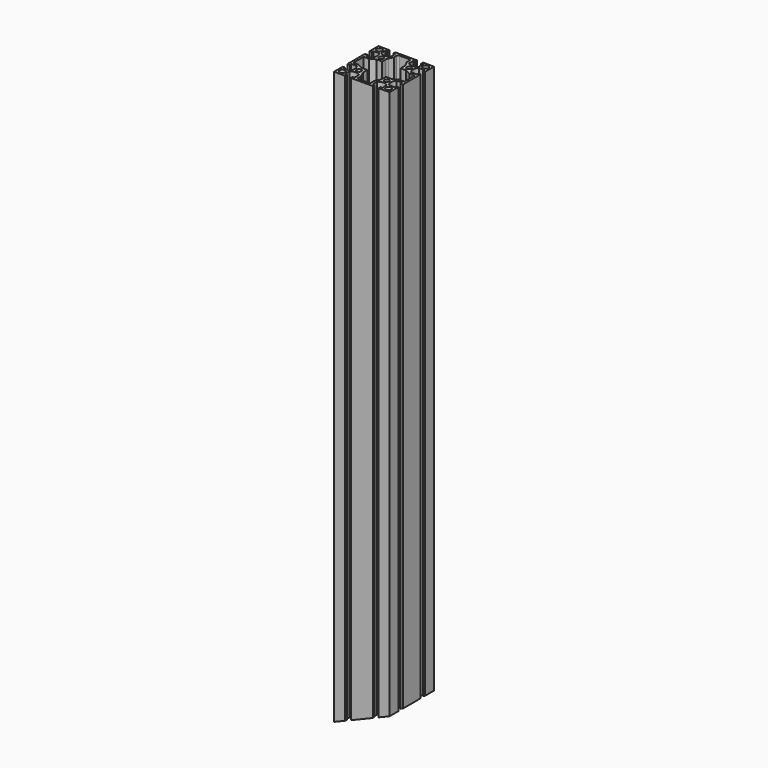
from build123d import *

# Parameters (mm, degrees)
F0_R          = 3
F0_R_2        = 2.5
F1_DEPTH      = 618.33
F2_R          = 2
F3_R          = 7
F5_DEPTH      = 30
F5_DEPTH_BACK = 30


# Not quite as in the source:
# - a feature names something its author has since deleted; it is built from what else it names


with BuildPart() as f1:
    # F0 (on Top) → F1 (new body)
    with BuildSketch(Plane.XY):
        with BuildLine():
            Line((18.15, -30), (30, -30))
            Line((30, -30), (30, -18.15))
            Line((30, -18.15), (27.5, -18.15))
            Line((27.5, -18.15), (27.5, -20.15))
            Line((27.5, -20.15), (21.5477069044, -20.15))
            ThreePointArc((21.5477069044, -20.15), (19.5, -15), (21.5477069044, -9.85))
            Line((21.5477069044, -9.85), (27.5, -9.85))
            Line((27.5, -9.85), (27.5, -11.85))
            Line((27.5, -11.85), (30, -11.85))
            Line((30, -11.85), (30, 11.85))
            Line((30, 11.85), (27.5, 11.85))
            Line((27.5, 11.85), (27.5, 9.85))
            Line((27.5, 9.85), (21.5477069044, 9.85))
            ThreePointArc((21.5477069044, 9.85), (19.5, 15), (21.5477069044, 20.15))
            Line((21.5477069044, 20.15), (27.5, 20.15))
            Line((27.5, 20.15), (27.5, 18.15))
            Line((27.5, 18.15), (30, 18.15))
            Line((30, 18.15), (30, 30))
            Line((30, 30), (18.15, 30))
            Line((18.15, 30), (18.15, 27.5))
            Line((18.15, 27.5), (20.15, 27.5))
            Line((20.15, 27.5), (20.15, 21.5477069044))
            ThreePointArc((20.15, 21.5477069044), (15, 19.5), (9.85, 21.5477069044))
            Line((9.85, 21.5477069044), (9.85, 27.5))
            Line((9.85, 27.5), (11.85, 27.5))
            Line((11.85, 27.5), (11.85, 30))
            Line((11.85, 30), (-11.85, 30))
            Line((-11.85, 30), (-11.85, 27.5))
            Line((-11.85, 27.5), (-9.85, 27.5))
            Line((-9.85, 27.5), (-9.85, 21.5477069044))
            ThreePointArc((-9.85, 21.5477069044), (-15, 19.5), (-20.15, 21.5477069044))
            Line((-20.15, 21.5477069044), (-20.15, 27.5))
            Line((-20.15, 27.5), (-18.15, 27.5))
            Line((-18.15, 27.5), (-18.15, 30))
            Line((-18.15, 30), (-30, 30))
            Line((-30, 30), (-30, 18.15))
            Line((-30, 18.15), (-27.5, 18.15))
            Line((-27.5, 18.15), (-27.5, 20.15))
            Line((-27.5, 20.15), (-21.5477069044, 20.15))
            ThreePointArc((-21.5477069044, 20.15), (-19.5, 15), (-21.5477069044, 9.85))
            Line((-21.5477069044, 9.85), (-27.5, 9.85))
            Line((-27.5, 9.85), (-27.5, 11.85))
            Line((-27.5, 11.85), (-30, 11.85))
            Line((-30, 11.85), (-30, -11.85))
            Line((-30, -11.85), (-27.5, -11.85))
            Line((-27.5, -11.85), (-27.5, -9.85))
            Line((-27.5, -9.85), (-21.5477069044, -9.85))
            ThreePointArc((-21.5477069044, -9.85), (-19.5, -15), (-21.5477069044, -20.15))
            Line((-21.5477069044, -20.15), (-27.5, -20.15))
            Line((-27.5, -20.15), (-27.5, -18.15))
            Line((-27.5, -18.15), (-30, -18.15))
            Line((-30, -18.15), (-30, -30))
            Line((-30, -30), (-18.15, -30))
            Line((-18.15, -30), (-18.15, -27.5))
            Line((-18.15, -27.5), (-20.15, -27.5))
            Line((-20.15, -27.5), (-20.15, -21.5477069044))
            ThreePointArc((-20.15, -21.5477069044), (-15, -19.5), (-9.85, -21.5477069044))
            Line((-9.85, -21.5477069044), (-9.85, -27.5))
            Line((-9.85, -27.5), (-11.85, -27.5))
            Line((-11.85, -27.5), (-11.85, -30))
            Line((-11.85, -30), (11.85, -30))
            Line((11.85, -30), (11.85, -27.5))
            Line((11.85, -27.5), (9.85, -27.5))
            Line((9.85, -27.5), (9.85, -21.5477069044))
            ThreePointArc((9.85, -21.5477069044), (15, -19.5), (20.15, -21.5477069044))
            Line((20.15, -21.5477069044), (20.15, -27.5))
            Line((20.15, -27.5), (18.15, -27.5))
            Line((18.15, -27.5), (18.15, -30))
        make_face()
        with Locations((-25, -25)):
            Circle(F0_R, mode=Mode.SUBTRACT)
        with Locations((-15, -15)):
            Circle(F0_R_2, mode=Mode.SUBTRACT)
        with Locations((25, -25)):
            Circle(F0_R, mode=Mode.SUBTRACT)
        with Locations((15, -15)):
            Circle(F0_R_2, mode=Mode.SUBTRACT)
        with Locations((-25, 25)):
            Circle(F0_R, mode=Mode.SUBTRACT)
        with Locations((-15, 15)):
            Circle(F0_R_2, mode=Mode.SUBTRACT)
        Polygon((-7, 22), (-7, 27.5), (0, 27.5), (7, 27.5), (7, 22), (10, 16), (10, 10), (16, 10), (22, 7), (27.5, 7), (27.5, 0), (27.5, -7), (22, -7), (16, -10), (10, -10), (10, -16), (7, -22), (7, -27.5), (0, -27.5), (-7, -27.5), (-7, -22), (-10, -16), (-10, -10), (-16, -10), (-22, -7), (-27.5, -7), (-27.5, 0), (-27.5, 7), (-22, 7), (-16, 10), (-10, 10), (-10, 16), align=None, mode=Mode.SUBTRACT)
        with Locations((15, 15)):
            Circle(F0_R_2, mode=Mode.SUBTRACT)
        with Locations((25, 25)):
            Circle(F0_R, mode=Mode.SUBTRACT)
    extrude(amount=F1_DEPTH)

    # F2
    f2_edges = [f1.edges().sort_by_distance(p)[0] for p in [
        (-7, 27.5, 309.165),
        (7, 27.5, 309.165),
    ]]
    fillet(f2_edges, radius=F2_R)

    # F3
    f3_edges = [f1.edges().sort_by_distance(p)[0] for p in [
        (-10, 16, 309.165),
        (10, 16, 309.165),
    ]]
    fillet(f3_edges, radius=F3_R)

    # F4 (on Front) → F5 (cut, two sides)
    with BuildSketch(Plane.XZ) as f5_sk:
        Polygon((227.6837248597, 106.7360936397), (-30, 0), (35.1751396755, -157.3467061341), (292.8588645352, -50.6106124944), align=None)
    extrude(amount=F5_DEPTH, mode=Mode.SUBTRACT)
    extrude(f5_sk.sketch, amount=-F5_DEPTH_BACK, mode=Mode.SUBTRACT)


solid = f1.part
